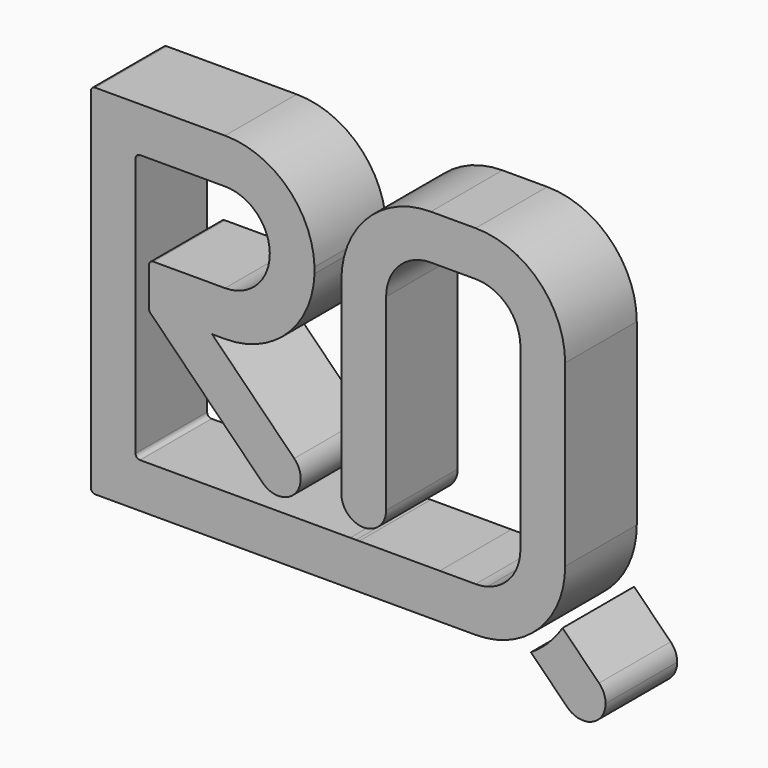
from build123d import *

# Parameters (mm, degrees)
F1_DEPTH = 10


# Not quite as in the source:
# - ends of sketch curves that miss each other by under 0.0002 mm in the source are joined


with BuildPart() as f1:
    # F0 (on Front) → F1 (new body)
    with BuildSketch(Plane.XZ):
        with BuildLine():
            Line((-25, -14.4999996647), (-25, 14.5))
            ThreePointArc((-25, 14.5), (-24.8535533906, 14.8535533906), (-24.5, 15))
            Line((-24.5, 15), (-15, 15))
            ThreePointArc((-15, 15), (-11.493877298, 13.5647024558), (-10.0006863175, 10.0828414395))
            ThreePointArc((-10.0006863175, 10.0828414395), (-11.4352975442, 6.493877298), (-15, 5))
            Line((-15, 5), (-23, 5))
            ThreePointArc((-23, 5), (-23.3535533906, 4.8535533906), (-23.5, 4.5))
            Line((-23.5, 4.5), (-23.5, 0.2061669839))
            ThreePointArc((-23.5, 0.2061669839), (-23.4887525914, 0.1007112853), (-23.4555163825, 0))
            Line((-23.4555163825, 0), (-16.4515272404, 0))
            Line((-16.4515272404, 0), (-15, 0))
            ThreePointArc((-15, 0), (-8.0470582749, 2.8127473004), (-5.0054901633, 9.6686797265))
            Line((-5.0054901633, 9.6686797265), (-5.0054901633, 10.3313202735))
            ThreePointArc((-5.0054901633, 10.3313202735), (-8.0470582749, 17.1872526996), (-15, 20))
            Line((-15, 20), (-25, 20))
            Line((-25, 20), (-29.5000011921, 20))
            ThreePointArc((-29.5000011921, 20), (-29.8535545827, 19.8535533906), (-30.0000011921, 19.5))
            Line((-30.0000011921, 19.5), (-30.0000011921, 17.5))
            Line((-30.0000011921, 17.5), (-30.0000011921, -19.5))
            ThreePointArc((-30.0000011921, -19.5), (-29.8535545827, -19.8535533906), (-29.5000011921, -20))
            Line((-29.5000011921, -20), (-25, -20))
            Line((-25, -20), (-2.0054901633, -20))
            Line((-2.0054901633, -20), (-0.3755952516, -20))
            Line((-0.3755952516, -20), (8.9945098367, -20))
            Line((8.9945098367, -20), (12.9945098367, -20))
            ThreePointArc((12.9945098367, -20), (16.8213441604, -19.2387953251), (20.0655776486, -17.0710678119))
            ThreePointArc((20.0655776486, -17.0710678119), (22.2333051618, -13.8268343237), (22.9945098367, -10))
            Line((22.9945098367, -10), (22.9945098367, 10))
            ThreePointArc((22.9945098367, 10), (20.0655776486, 17.0710678119), (12.9945098367, 20))
            Line((12.9945098367, 20), (7.9945098367, 20))
            ThreePointArc((7.9945098367, 20), (0.9234420249, 17.0710678119), (-2.0054901633, 10))
            Line((-2.0054901633, 10), (-2.0054901633, -11.0000000643))
            ThreePointArc((-2.0054901633, -11.0000000643), (-1.2732571162, -12.7677670173), (0.4945098367, -13.5000000643))
            ThreePointArc((0.4945098367, -13.5000000643), (2.262277125, -12.7677670173), (2.994510172, -11.0000000643))
            Line((2.994510172, -11.0000000643), (2.994510172, 10))
            ThreePointArc((2.994510172, 10), (4.4589761679, 13.5355336689), (7.9945098367, 14.9999996647))
            Line((7.9945098367, 14.9999996647), (12.9945098367, 14.9999996647))
            ThreePointArc((12.9945098367, 14.9999996647), (16.5300435056, 13.5355336689), (17.9945095014, 10))
            Line((17.9945095014, 10), (17.9945095014, -10))
            ThreePointArc((17.9945095014, -10), (16.9612762133, -13.0438070177), (14.2886047885, -14.8296288577))
            ThreePointArc((14.2886047885, -14.8296288577), (13.6471406581, -14.9572239871), (12.9945098367, -14.9999996647))
            Line((12.9945098367, -14.9999996647), (8.9945098367, -14.9999996647))
            Line((8.9945098367, -14.9999996647), (-0.0054901633, -15.0000000878))
            Line((-0.0054901633, -15.0000000878), (-0.3755952516, -15.0000001052))
            Line((-0.3755952516, -15.0000001052), (-1.0054901633, -15.0000001348))
            Line((-1.0054901633, -15.0000001348), (-24.5, -14.9999996647))
            ThreePointArc((-24.5, -14.9999996647), (-24.8535533906, -14.8535530553), (-25, -14.4999996647))
        make_face()
        with BuildLine():
            Line((-16.4515272404, 0), (-23.4555163825, 0))
            ThreePointArc((-23.4555163825, 0), (-23.4116485183, -0.0776384025), (-23.3546867552, -0.1462493971))
            Line((-23.3546867552, -0.1462493971), (-10.8196093867, -12.7620815701))
            ThreePointArc((-10.8196093867, -12.7620815701), (-9.0542025953, -13.4999867782), (-7.284093705, -12.773433441))
            ThreePointArc((-7.284093705, -12.773433441), (-6.5461885926, -11.0080267446), (-7.2727419298, -9.2379178544))
            Line((-7.2727419298, -9.2379178544), (-16.4515272404, 0))
        make_face()
    extrude(amount=-F1_DEPTH)


with BuildPart() as f1b:
    # F0 (on Front) → F1, piece 2 (new body)
    with BuildSketch(Plane.XZ):
        with BuildLine():
            ThreePointArc((26.7830920699, -20.2530483272), (25.0153251169, -19.5208152802), (23.2475581639, -20.2530483272))
            ThreePointArc((23.2475581639, -20.2530483272), (22.5153251169, -22.0208152802), (23.2475581639, -23.7885822331))
            ThreePointArc((23.2475581639, -23.7885822331), (25.9720336978, -24.3305141114), (27.5153251169, -22.0208152802))
            ThreePointArc((27.5153251169, -22.0208152802), (27.3250239482, -21.0641066993), (26.7830920699, -20.2530483272))
        make_face()
        with BuildLine():
            Line((21.1262378204, -18.1317279836), (22.9945098367, -20))
            Line((22.9945098367, -20), (23.2475581639, -20.2530483272))
            ThreePointArc((23.2475581639, -20.2530483272), (25.0153251169, -19.5208152802), (26.7830920699, -20.2530483272))
            Line((26.7830920699, -20.2530483272), (22.6995307229, -16.1694869802))
            ThreePointArc((22.6995307229, -16.1694869802), (21.9666890592, -17.193747285), (21.1262378204, -18.1317279836))
        make_face()
        with BuildLine():
            Line((19.4589759308, -20), (22.9945098367, -20))
            Line((22.9945098367, -20), (21.1262378204, -18.1317279836))
            ThreePointArc((21.1262378204, -18.1317279836), (20.1882571217, -18.9721792225), (19.163996817, -19.7050208862))
            Line((19.163996817, -19.7050208862), (19.4589759308, -20))
        make_face()
        with BuildLine():
            Line((23.2475581639, -20.2530483272), (22.9945098367, -20))
            Line((22.9945098367, -20), (19.4589759308, -20))
            Line((19.4589759308, -20), (23.2475581639, -23.7885822331))
            ThreePointArc((23.2475581639, -23.7885822331), (22.5153251169, -22.0208152802), (23.2475581639, -20.2530483272))
        make_face()
    extrude(amount=-F1_DEPTH)


solid = Compound([f1.part, f1b.part])
